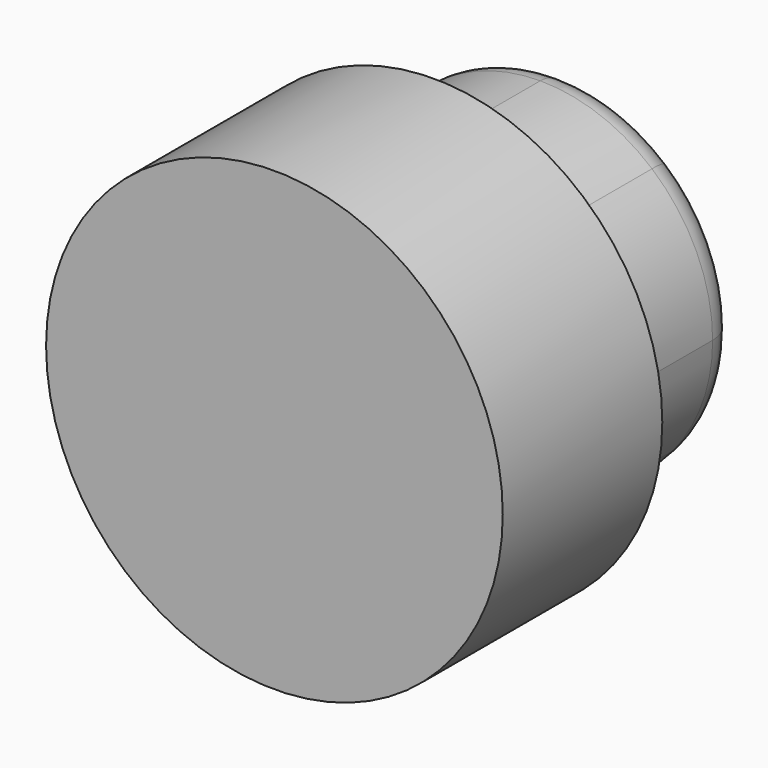
from build123d import *

# Parameters (mm, degrees)
F0_R          = 35.5650763439
F1_DEPTH      = 76.2
F1_DEPTH_BACK = 63.5
F2_R          = 12.7
F3_SIZE       = 7.62
F4_DEPTH      = 177.8
F5_R          = 87.2500629337
F6_DEPTH      = 152.4
F7_DEPTH      = 76.2


# Not quite as in the source:
# - the program builds the solid bodies; features that only make, move or delete a surface that nothing else refers to are left out


with BuildPart() as f1:
    # F0 (on Front) → F1 (new body, two sides)
    with BuildSketch(Plane.XZ) as f1_sk:
        with BuildLine():
            Line((-39.0193847966, 40.3927160345), (-45.8709552438, 47.2442864817))
            ThreePointArc((-45.8709552438, 47.2442864817), (-60.649609484, 25.6474562011), (-65.8495796505, 0))
            Line((-65.8495796505, 0), (-56.161231277, 0))
            ThreePointArc((-56.161231277, 0), (-51.6984554527, 21.9397721581), (-39.0193847966, 40.3927160345))
        make_face()
        with BuildLine():
            Line((0, 56.161231277), (0, 65.8495796505))
            ThreePointArc((0, 65.8495796505), (-24.7502599425, 61.0212403424), (-45.8709552438, 47.2442864817))
            Line((-45.8709552438, 47.2442864817), (-39.0193847966, 40.3927160345))
            ThreePointArc((-39.0193847966, 40.3927160345), (-21.0425667568, 52.0700900982), (0, 56.161231277))
        make_face()
        with BuildLine():
            Line((35.8053838633, 43.2672900116), (42.6820145021, 50.1439206504))
            ThreePointArc((42.6820145021, 50.1439206504), (22.7399543018, 61.7985567671), (0, 65.8495796505))
            Line((0, 65.8495796505), (0, 56.161231277))
            ThreePointArc((0, 56.161231277), (19.0281320349, 52.8395125811), (35.8053838633, 43.2672900116))
        make_face()
        with BuildLine():
            Line((56.161231277, 0), (65.8495796505, 0))
            ThreePointArc((65.8495796505, 0), (59.7777544482, 27.6186026669), (42.6820145021, 50.1439206504))
            Line((42.6820145021, 50.1439206504), (35.8053838633, 43.2672900116))
            ThreePointArc((35.8053838633, 43.2672900116), (50.8180988559, 23.9082564655), (56.161231277, 0))
        make_face()
        with BuildLine():
            ThreePointArc((50.469556702, -42.2964654133), (61.8852415125, -22.5029780938), (65.8495796505, 0))
            Line((65.8495796505, 0), (56.161231277, 0))
            ThreePointArc((56.161231277, 0), (52.9245852031, -18.7902149969), (43.5877113736, -35.4146200849))
            Line((43.5877113736, -35.4146200849), (50.469556702, -42.2964654133))
        make_face()
        with BuildLine():
            ThreePointArc((0, -65.8495796505), (27.8474655219, -59.6714823358), (50.469556702, -42.2964654133))
            Line((50.469556702, -42.2964654133), (43.5877113736, -35.4146200849))
            ThreePointArc((43.5877113736, -35.4146200849), (24.1366446443, -50.7100215328), (0, -56.161231277))
            Line((0, -56.161231277), (0, -65.8495796505))
        make_face()
        with BuildLine():
            ThreePointArc((-46.445321126, -46.6797524163), (-25.1229483276, -60.8687490218), (0, -65.8495796505))
            Line((0, -65.8495796505), (0, -56.161231277))
            ThreePointArc((0, -56.161231277), (-21.4153744517, -51.9178739514), (-39.5945988408, -39.8290301311))
            Line((-39.5945988408, -39.8290301311), (-46.445321126, -46.6797524163))
        make_face()
        with BuildLine():
            ThreePointArc((-65.8495796505, 0), (-60.8053123215, -25.2760980698), (-46.445321126, -46.6797524163))
            Line((-46.445321126, -46.6797524163), (-39.5945988408, -39.8290301311))
            ThreePointArc((-39.5945988408, -39.8290301311), (-51.8544372323, -21.5685242394), (-56.161231277, 0))
            Line((-56.161231277, 0), (-65.8495796505, 0))
        make_face()
        with BuildLine():
            ThreePointArc((43.5877113736, -35.4146200849), (52.9245852031, -18.7902149969), (56.161231277, 0))
            ThreePointArc((56.161231277, 0), (50.8180988559, 23.9082564655), (35.8053838633, 43.2672900116))
            ThreePointArc((35.8053838633, 43.2672900116), (19.0281320349, 52.8395125811), (0, 56.161231277))
            ThreePointArc((0, 56.161231277), (-21.0425667568, 52.0700900982), (-39.0193847966, 40.3927160345))
            ThreePointArc((-39.0193847966, 40.3927160345), (-51.6984554527, 21.9397721581), (-56.161231277, 0))
            ThreePointArc((-56.161231277, 0), (-51.8544372323, -21.5685242394), (-39.5945988408, -39.8290301311))
            ThreePointArc((-39.5945988408, -39.8290301311), (-21.4153744517, -51.9178739514), (0, -56.161231277))
            ThreePointArc((0, -56.161231277), (24.1366446443, -50.7100215328), (43.5877113736, -35.4146200849))
        make_face()
        Circle(F0_R, mode=Mode.SUBTRACT)
    extrude(amount=F1_DEPTH)
    extrude(f1_sk.sketch, amount=-F1_DEPTH_BACK)

    # F2
    f2_edges = [f1.edges().sort_by_distance(p)[0] for p in [
        (65.84958, -76.2, 0),
        (65.84958, 63.5, 0),
    ]]
    fillet(f2_edges, radius=F2_R)

    # F3
    f3_edges = [f1.edges().sort_by_distance(p)[0] for p in [
        (-35.565076, -76.2, 0),
        (-35.565076, 63.5, 0),
    ]]
    chamfer(f3_edges, length=F3_SIZE)

    # F4 (cut): a face of the model
    f4_faces = [f1.faces().sort_by_distance(p)[0] for p in [
        (-44.6883734714, 63.5, 0),
    ]]
    extrude(f4_faces, amount=-F4_DEPTH, mode=Mode.SUBTRACT)


with BuildPart() as f6:
    # F5 (on Front) → F6 (new body)
    with BuildSketch(Plane.XZ):
        Circle(F5_R)
    extrude(amount=F6_DEPTH)

    # F7 (cut): a face of the model
    f7_faces = [f6.faces().sort_by_distance(p)[0] for p in [
        (0, -152.4, 0),
    ]]
    extrude(f7_faces, amount=-F7_DEPTH, mode=Mode.SUBTRACT)


solid = Compound([f1.part, f6.part])
